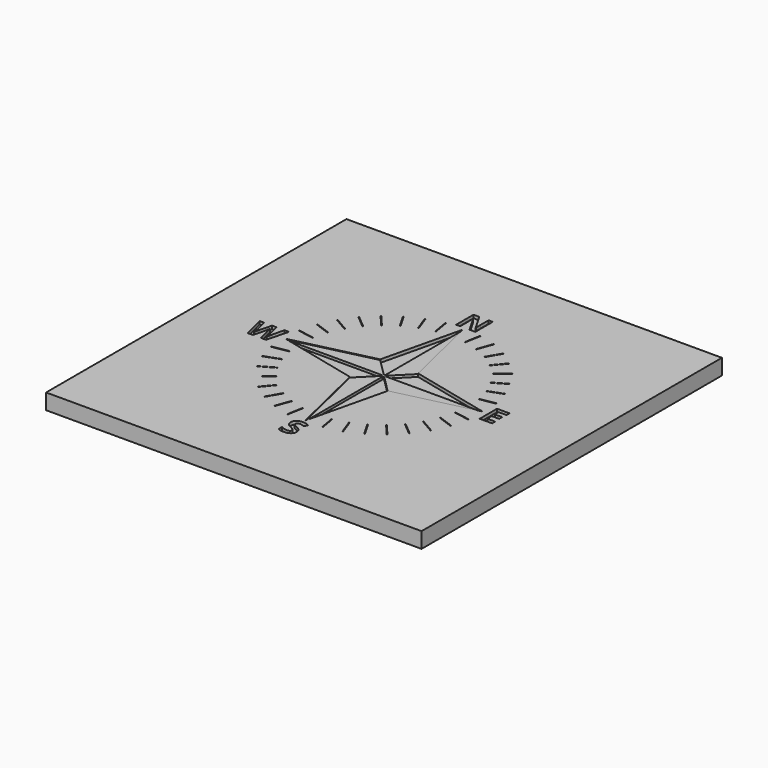
from build123d import *

# Parameters (mm, degrees)
F0_W         = 152.4
F0_H         = 152.4
F1_DEPTH     = 6.35
F2_TEXT_SIZE = 12.3472222222
F3_DEPTH     = 1.27
F5_DEPTH     = 1.27
F7_DEPTH     = 1.016
F9_DEPTH     = 1.27


# Not quite as in the source:
# - Text() gives the source's letters only with a copy of the font that has no kerning and outlines rounded to 1/6400 em; it was checked with that copy


with BuildPart() as f1:
    # F0 (on Top) → F1 (new body)
    with BuildSketch(Plane.XY):
        with Locations((76.2, 76.2)):
            Rectangle(F0_W, F0_H)
    extrude(amount=F1_DEPTH)

    # F2 (on face) → F3 (cut)
    with BuildSketch(Plane.XY.offset(6.35)):
        with Locations((71.3353873698, 117.475)):
            Text('N', F2_TEXT_SIZE, font='Open Sans', font_style=FontStyle.BOLD, text_align=(TextAlign.LEFT, TextAlign.BOTTOM))
        with Locations((117.475, 71.755)):
            Text('E', F2_TEXT_SIZE, font='Open Sans', font_style=FontStyle.BOLD, text_align=(TextAlign.LEFT, TextAlign.BOTTOM))
        with Locations((72.643421224, 26.035)):
            Text('S', F2_TEXT_SIZE, font='Open Sans', font_style=FontStyle.BOLD, text_align=(TextAlign.LEFT, TextAlign.BOTTOM))
        with Locations((22.1861393229, 71.755)):
            Text('W', F2_TEXT_SIZE, font='Open Sans', font_style=FontStyle.BOLD, text_align=(TextAlign.LEFT, TextAlign.BOTTOM))
    extrude(amount=-F3_DEPTH, mode=Mode.SUBTRACT)

    # F4 (on face) → F5 (cut)
    with BuildSketch(Plane.XY.offset(6.35)):
        Polygon((83.8932692308, 68.5067307692), (116.205, 76.2), (83.8932692308, 83.8932692308), (76.2, 116.205), (68.5067307692, 83.8932692308), (36.195, 76.2), (68.5067307692, 68.5067307692), (76.2, 36.195), align=None)
    extrude(amount=-F5_DEPTH, mode=Mode.SUBTRACT)

    # F6 (on face) → F7 (join)
    with BuildSketch(Plane.XY.offset(5.08)):
        with BuildLine():
            Line((83.8932692308, 83.8932692308), (76.2, 116.205))
            Line((76.2, 116.205), (76.2, 76.962))
            ThreePointArc((76.2, 76.962), (76.4916047755, 76.9039962038), (76.7388153673, 76.7388153673))
            Line((76.7388153673, 76.7388153673), (83.8932692308, 83.8932692308))
        make_face()
        with BuildLine():
            Line((68.5067307692, 83.8932692308), (36.195, 76.2))
            Line((36.195, 76.2), (75.438, 76.2))
            ThreePointArc((75.438, 76.2), (75.4960037962, 76.4916047755), (75.6611846327, 76.7388153673))
            Line((75.6611846327, 76.7388153673), (68.5067307692, 83.8932692308))
        make_face()
        with BuildLine():
            Line((75.6611846327, 75.6611846327), (68.5067307692, 68.5067307692))
            Line((68.5067307692, 68.5067307692), (76.2, 36.195))
            Line((76.2, 36.195), (76.2, 75.438))
            ThreePointArc((76.2, 75.438), (75.9083952245, 75.4960037962), (75.6611846327, 75.6611846327))
        make_face()
        with BuildLine():
            Line((76.7388153673, 75.6611846327), (83.8932692308, 68.5067307692))
            Line((83.8932692308, 68.5067307692), (116.205, 76.2))
            Line((116.205, 76.2), (76.962, 76.2))
            ThreePointArc((76.962, 76.2), (76.9039962038, 75.9083952245), (76.7388153673, 75.6611846327))
        make_face()
        with BuildLine():
            ThreePointArc((75.438, 76.2), (75.4960037962, 75.9083952245), (75.6611846327, 75.6611846327))
            ThreePointArc((75.6611846327, 75.6611846327), (75.9083952245, 75.4960037962), (76.2, 75.438))
            ThreePointArc((76.2, 75.438), (76.4916047755, 75.4960037962), (76.7388153673, 75.6611846327))
            ThreePointArc((76.7388153673, 75.6611846327), (76.9039962038, 75.9083952245), (76.962, 76.2))
            ThreePointArc((76.962, 76.2), (76.9039962038, 76.4916047755), (76.7388153673, 76.7388153673))
            ThreePointArc((76.7388153673, 76.7388153673), (76.4916047755, 76.9039962038), (76.2, 76.962))
            ThreePointArc((76.2, 76.962), (75.9083952245, 76.9039962038), (75.6611846327, 76.7388153673))
            ThreePointArc((75.6611846327, 76.7388153673), (75.4960037962, 76.4916047755), (75.438, 76.2))
        make_face()
    extrude(amount=F7_DEPTH)

    # F8 (on face) → F9 (cut)
    with BuildSketch(Plane.XY.offset(6.35)):
        with BuildLine():
            Line((83.1301044375, 116.233939156), (82.0274385094, 109.9804099244))
            ThreePointArc((82.0274385094, 109.9804099244), (82.1304557754, 109.8332860212), (82.2775796786, 109.9363032873))
            Line((82.2775796786, 109.9363032873), (83.3802456068, 116.1898325189))
            ThreePointArc((83.3802456068, 116.1898325189), (83.2772283407, 116.3369564221), (83.1301044375, 116.233939156))
        make_face()
        with BuildLine():
            Line((89.9766411586, 114.4223336579), (87.8048132484, 108.4552855159))
            ThreePointArc((87.8048132484, 108.4552855159), (87.8807176531, 108.2925079948), (88.0434951741, 108.3684123995))
            Line((88.0434951741, 108.3684123995), (90.2153230842, 114.3354605415))
            ThreePointArc((90.2153230842, 114.3354605415), (90.1394186796, 114.4982380625), (89.9766411586, 114.4223336579))
        make_face()
        with BuildLine():
            Line((96.4045816093, 111.4493618929), (93.2295816093, 105.9501005789))
            ThreePointArc((93.2295816093, 105.9501005789), (93.2760668356, 105.7766153526), (93.4495520618, 105.8231005789))
            Line((93.4495520618, 105.8231005789), (96.6245520618, 111.3223618929))
            ThreePointArc((96.6245520618, 111.3223618929), (96.5780668356, 111.4958471192), (96.4045816093, 111.4493618929))
        make_face()
        with BuildLine():
            Line((102.2186160718, 107.4053561039), (98.1369147503, 102.5409738901))
            ThreePointArc((98.1369147503, 102.5409738901), (98.1525683681, 102.3620522194), (98.3314900389, 102.3777058373))
            Line((98.3314900389, 102.3777058373), (102.4131913604, 107.2420880511))
            ThreePointArc((102.4131913604, 107.2420880511), (102.3975377425, 107.4210097218), (102.2186160718, 107.4053561039))
        make_face()
        with BuildLine():
            Line((107.2420880511, 102.4131913604), (102.3777058373, 98.3314900389))
            ThreePointArc((102.3777058373, 98.3314900389), (102.3620522194, 98.1525683681), (102.5409738901, 98.1369147503))
            Line((102.5409738901, 98.1369147503), (107.4053561039, 102.2186160718))
            ThreePointArc((107.4053561039, 102.2186160718), (107.4210097218, 102.3975377425), (107.2420880511, 102.4131913604))
        make_face()
        with BuildLine():
            Line((111.3223618929, 96.6245520618), (105.8231005789, 93.4495520618))
            ThreePointArc((105.8231005789, 93.4495520618), (105.7766153526, 93.2760668356), (105.9501005789, 93.2295816093))
            Line((105.9501005789, 93.2295816093), (111.4493618929, 96.4045816093))
            ThreePointArc((111.4493618929, 96.4045816093), (111.4958471192, 96.5780668356), (111.3223618929, 96.6245520618))
        make_face()
        with BuildLine():
            Line((114.3354605415, 90.2153230842), (108.3684123995, 88.0434951741))
            ThreePointArc((108.3684123995, 88.0434951741), (108.2925079948, 87.8807176531), (108.4552855159, 87.8048132484))
            Line((108.4552855159, 87.8048132484), (114.4223336579, 89.9766411586))
            ThreePointArc((114.4223336579, 89.9766411586), (114.4982380625, 90.1394186796), (114.3354605415, 90.2153230842))
        make_face()
        with BuildLine():
            Line((116.1898325189, 83.3802456068), (109.9363032873, 82.2775796786))
            ThreePointArc((109.9363032873, 82.2775796786), (109.8332860212, 82.1304557754), (109.9804099244, 82.0274385094))
            Line((109.9804099244, 82.0274385094), (116.233939156, 83.1301044375))
            ThreePointArc((116.233939156, 83.1301044375), (116.3369564221, 83.2772283407), (116.1898325189, 83.3802456068))
        make_face()
        with BuildLine():
            Line((116.233939156, 69.2698955625), (109.9804099244, 70.3725614906))
            ThreePointArc((109.9804099244, 70.3725614906), (109.8332860212, 70.2695442246), (109.9363032873, 70.1224203214))
            Line((109.9363032873, 70.1224203214), (116.1898325189, 69.0197543932))
            ThreePointArc((116.1898325189, 69.0197543932), (116.3369564221, 69.1227716593), (116.233939156, 69.2698955625))
        make_face()
        with BuildLine():
            Line((114.4223336579, 62.4233588414), (108.4552855159, 64.5951867516))
            ThreePointArc((108.4552855159, 64.5951867516), (108.2925079948, 64.5192823469), (108.3684123995, 64.3565048259))
            Line((108.3684123995, 64.3565048259), (114.3354605415, 62.1846769158))
            ThreePointArc((114.3354605415, 62.1846769158), (114.4982380625, 62.2605813204), (114.4223336579, 62.4233588414))
        make_face()
        with BuildLine():
            Line((111.4493618929, 55.9954183907), (105.9501005789, 59.1704183907))
            ThreePointArc((105.9501005789, 59.1704183907), (105.7766153526, 59.1239331644), (105.8231005789, 58.9504479382))
            Line((105.8231005789, 58.9504479382), (111.3223618929, 55.7754479382))
            ThreePointArc((111.3223618929, 55.7754479382), (111.4958471192, 55.8219331644), (111.4493618929, 55.9954183907))
        make_face()
        with BuildLine():
            Line((107.4053561039, 50.1813839282), (102.5409738901, 54.2630852497))
            ThreePointArc((102.5409738901, 54.2630852497), (102.3620522194, 54.2474316319), (102.3777058373, 54.0685099611))
            Line((102.3777058373, 54.0685099611), (107.2420880511, 49.9868086396))
            ThreePointArc((107.2420880511, 49.9868086396), (107.4210097218, 50.0024622575), (107.4053561039, 50.1813839282))
        make_face()
        with BuildLine():
            Line((102.4131913604, 45.1579119489), (98.3314900389, 50.0222941627))
            ThreePointArc((98.3314900389, 50.0222941627), (98.1525683681, 50.0379477806), (98.1369147503, 49.8590261099))
            Line((98.1369147503, 49.8590261099), (102.2186160718, 44.9946438961))
            ThreePointArc((102.2186160718, 44.9946438961), (102.3975377425, 44.9789902782), (102.4131913604, 45.1579119489))
        make_face()
        with BuildLine():
            Line((96.6245520618, 41.0776381071), (93.4495520618, 46.5768994211))
            ThreePointArc((93.4495520618, 46.5768994211), (93.2760668356, 46.6233846474), (93.2295816093, 46.4498994211))
            Line((93.2295816093, 46.4498994211), (96.4045816093, 40.9506381071))
            ThreePointArc((96.4045816093, 40.9506381071), (96.5780668356, 40.9041528808), (96.6245520618, 41.0776381071))
        make_face()
        with BuildLine():
            Line((90.2153230842, 38.0645394585), (88.0434951741, 44.0315876005))
            ThreePointArc((88.0434951741, 44.0315876005), (87.8807176531, 44.1074920052), (87.8048132484, 43.9447144841))
            Line((87.8048132484, 43.9447144841), (89.9766411586, 37.9776663421))
            ThreePointArc((89.9766411586, 37.9776663421), (90.1394186796, 37.9017619375), (90.2153230842, 38.0645394585))
        make_face()
        with BuildLine():
            Line((83.3802456068, 36.2101674811), (82.2775796786, 42.4636967127))
            ThreePointArc((82.2775796786, 42.4636967127), (82.1304557754, 42.5667139788), (82.0274385094, 42.4195900756))
            Line((82.0274385094, 42.4195900756), (83.1301044375, 36.166060844))
            ThreePointArc((83.1301044375, 36.166060844), (83.2772283407, 36.0630435779), (83.3802456068, 36.2101674811))
        make_face()
        with BuildLine():
            Line((69.2698955625, 36.166060844), (70.3725614906, 42.4195900756))
            ThreePointArc((70.3725614906, 42.4195900756), (70.2695442246, 42.5667139788), (70.1224203214, 42.4636967127))
            Line((70.1224203214, 42.4636967127), (69.0197543932, 36.2101674811))
            ThreePointArc((69.0197543932, 36.2101674811), (69.1227716593, 36.0630435779), (69.2698955625, 36.166060844))
        make_face()
        with BuildLine():
            Line((62.4233588414, 37.9776663421), (64.5951867516, 43.9447144841))
            ThreePointArc((64.5951867516, 43.9447144841), (64.5192823469, 44.1074920052), (64.3565048259, 44.0315876005))
            Line((64.3565048259, 44.0315876005), (62.1846769158, 38.0645394585))
            ThreePointArc((62.1846769158, 38.0645394585), (62.2605813204, 37.9017619375), (62.4233588414, 37.9776663421))
        make_face()
        with BuildLine():
            Line((55.9954183907, 40.9506381071), (59.1704183907, 46.4498994211))
            ThreePointArc((59.1704183907, 46.4498994211), (59.1239331644, 46.6233846474), (58.9504479382, 46.5768994211))
            Line((58.9504479382, 46.5768994211), (55.7754479382, 41.0776381071))
            ThreePointArc((55.7754479382, 41.0776381071), (55.8219331644, 40.9041528808), (55.9954183907, 40.9506381071))
        make_face()
        with BuildLine():
            Line((50.1813839282, 44.9946438961), (54.2630852497, 49.8590261099))
            ThreePointArc((54.2630852497, 49.8590261099), (54.2474316319, 50.0379477806), (54.0685099611, 50.0222941627))
            Line((54.0685099611, 50.0222941627), (49.9868086396, 45.1579119489))
            ThreePointArc((49.9868086396, 45.1579119489), (50.0024622575, 44.9789902782), (50.1813839282, 44.9946438961))
        make_face()
        with BuildLine():
            Line((45.1579119489, 49.9868086396), (50.0222941627, 54.0685099611))
            ThreePointArc((50.0222941627, 54.0685099611), (50.0379477806, 54.2474316319), (49.8590261099, 54.2630852497))
            Line((49.8590261099, 54.2630852497), (44.9946438961, 50.1813839282))
            ThreePointArc((44.9946438961, 50.1813839282), (44.9789902782, 50.0024622575), (45.1579119489, 49.9868086396))
        make_face()
        with BuildLine():
            Line((41.0776381071, 55.7754479382), (46.5768994211, 58.9504479382))
            ThreePointArc((46.5768994211, 58.9504479382), (46.6233846474, 59.1239331644), (46.4498994211, 59.1704183907))
            Line((46.4498994211, 59.1704183907), (40.9506381071, 55.9954183907))
            ThreePointArc((40.9506381071, 55.9954183907), (40.9041528808, 55.8219331644), (41.0776381071, 55.7754479382))
        make_face()
        with BuildLine():
            Line((38.0645394585, 62.1846769158), (44.0315876005, 64.3565048259))
            ThreePointArc((44.0315876005, 64.3565048259), (44.1074920052, 64.5192823469), (43.9447144841, 64.5951867516))
            Line((43.9447144841, 64.5951867516), (37.9776663421, 62.4233588414))
            ThreePointArc((37.9776663421, 62.4233588414), (37.9017619375, 62.2605813204), (38.0645394585, 62.1846769158))
        make_face()
        with BuildLine():
            Line((36.2101674811, 69.0197543932), (42.4636967127, 70.1224203214))
            ThreePointArc((42.4636967127, 70.1224203214), (42.5667139788, 70.2695442246), (42.4195900756, 70.3725614906))
            Line((42.4195900756, 70.3725614906), (36.166060844, 69.2698955625))
            ThreePointArc((36.166060844, 69.2698955625), (36.0630435779, 69.1227716593), (36.2101674811, 69.0197543932))
        make_face()
        with BuildLine():
            Line((36.166060844, 83.1301044375), (42.4195900756, 82.0274385094))
            ThreePointArc((42.4195900756, 82.0274385094), (42.5667139788, 82.1304557754), (42.4636967127, 82.2775796786))
            Line((42.4636967127, 82.2775796786), (36.2101674811, 83.3802456068))
            ThreePointArc((36.2101674811, 83.3802456068), (36.0630435779, 83.2772283407), (36.166060844, 83.1301044375))
        make_face()
        with BuildLine():
            Line((37.9776663421, 89.9766411586), (43.9447144841, 87.8048132484))
            ThreePointArc((43.9447144841, 87.8048132484), (44.1074920052, 87.8807176531), (44.0315876005, 88.0434951741))
            Line((44.0315876005, 88.0434951741), (38.0645394585, 90.2153230842))
            ThreePointArc((38.0645394585, 90.2153230842), (37.9017619375, 90.1394186796), (37.9776663421, 89.9766411586))
        make_face()
        with BuildLine():
            Line((40.9506381071, 96.4045816093), (46.4498994211, 93.2295816093))
            ThreePointArc((46.4498994211, 93.2295816093), (46.6233846474, 93.2760668356), (46.5768994211, 93.4495520618))
            Line((46.5768994211, 93.4495520618), (41.0776381071, 96.6245520618))
            ThreePointArc((41.0776381071, 96.6245520618), (40.9041528808, 96.5780668356), (40.9506381071, 96.4045816093))
        make_face()
        with BuildLine():
            Line((44.9946438961, 102.2186160718), (49.8590261099, 98.1369147503))
            ThreePointArc((49.8590261099, 98.1369147503), (50.0379477806, 98.1525683681), (50.0222941627, 98.3314900389))
            Line((50.0222941627, 98.3314900389), (45.1579119489, 102.4131913604))
            ThreePointArc((45.1579119489, 102.4131913604), (44.9789902782, 102.3975377425), (44.9946438961, 102.2186160718))
        make_face()
        with BuildLine():
            Line((49.9868086396, 107.2420880511), (54.0685099611, 102.3777058373))
            ThreePointArc((54.0685099611, 102.3777058373), (54.2474316319, 102.3620522194), (54.2630852497, 102.5409738901))
            Line((54.2630852497, 102.5409738901), (50.1813839282, 107.4053561039))
            ThreePointArc((50.1813839282, 107.4053561039), (50.0024622575, 107.4210097218), (49.9868086396, 107.2420880511))
        make_face()
        with BuildLine():
            Line((55.7754479382, 111.3223618929), (58.9504479382, 105.8231005789))
            ThreePointArc((58.9504479382, 105.8231005789), (59.1239331644, 105.7766153526), (59.1704183907, 105.9501005789))
            Line((59.1704183907, 105.9501005789), (55.9954183907, 111.4493618929))
            ThreePointArc((55.9954183907, 111.4493618929), (55.8219331644, 111.4958471192), (55.7754479382, 111.3223618929))
        make_face()
        with BuildLine():
            Line((62.1846769158, 114.3354605415), (64.3565048259, 108.3684123995))
            ThreePointArc((64.3565048259, 108.3684123995), (64.5192823469, 108.2925079948), (64.5951867516, 108.4552855159))
            Line((64.5951867516, 108.4552855159), (62.4233588414, 114.4223336579))
            ThreePointArc((62.4233588414, 114.4223336579), (62.2605813204, 114.4982380625), (62.1846769158, 114.3354605415))
        make_face()
        with BuildLine():
            Line((69.0197543932, 116.1898325189), (70.1224203214, 109.9363032873))
            ThreePointArc((70.1224203214, 109.9363032873), (70.2695442246, 109.8332860212), (70.3725614906, 109.9804099244))
            Line((70.3725614906, 109.9804099244), (69.2698955625, 116.233939156))
            ThreePointArc((69.2698955625, 116.233939156), (69.1227716593, 116.3369564221), (69.0197543932, 116.1898325189))
        make_face()
    extrude(amount=-F9_DEPTH, mode=Mode.SUBTRACT)


solid = f1.part
